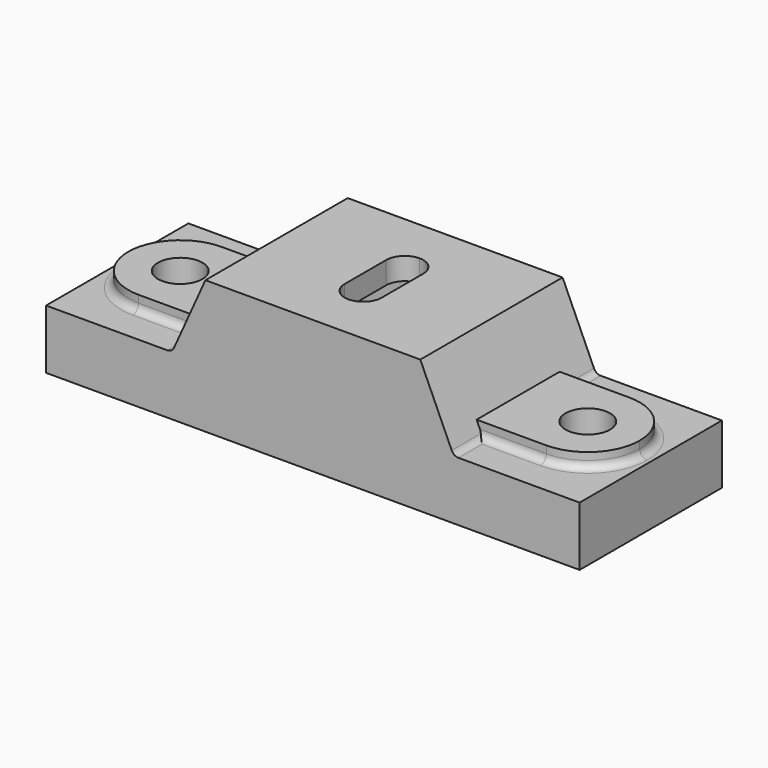
from build123d import *

# Parameters (mm, degrees)
F1_DEPTH  = 60
F3_DEPTH  = 25
F4_W      = 7.5
F4_H      = 10
F5_DEPTH  = 70
F6_R      = 34.99999
F7_R      = 5
F8_R      = 15
F9_DEPTH  = 50
F11_DEPTH = 90
F13_DEPTH = 45
F14_R     = 5


# Not quite as in the source:
# - a fillet or chamfer is up to 0.001 mm smaller than in the source, because OpenCascade refuses the exact size
# - a pattern or mirror of a feature is missing from the dataset's text; its kind, count and spacing are read off the source's solid


with BuildPart() as f1:
    # F0 (on Front) → F1 (new body, symmetric)
    with BuildSketch(Plane.XZ):
        Polygon((-180, 0), (0, 0), (180, 0), (180, 50), (90.5, 50), (72.5, 90), (0, 90), (-72.5, 90), (-90.5, 50), (-180, 50), align=None)
    extrude(amount=F1_DEPTH, both=True)

    # F2 (on face) → F3 (cut)
    with BuildSketch(Plane.XZ.offset(60)):
        Polygon((-95, 40), (-90.5, 50), (-180, 50), (-180, 40), align=None)
        Polygon((180, 50), (90.5, 50), (95, 40), (180, 40), align=None)
    f3 = extrude(amount=-F3_DEPTH, mode=Mode.SUBTRACT)

    # F3_copies: F3 across plane
    add(f3.mirror(Plane.ZX), mode=Mode.SUBTRACT)

    # F4 (on face) → F5 (cut)
    with BuildSketch(Plane.XZ.offset(35)):
        with Locations((-176.25, 45)):
            Rectangle(F4_W, F4_H)
        with Locations((176.25, 45)):
            Rectangle(F4_W, F4_H)
    extrude(amount=-F5_DEPTH, mode=Mode.SUBTRACT)

    # F6 (radius 35 in the source; OpenCascade refuses exactly that, so slightly less here)
    f6_edges = [f1.edges().sort_by_distance(p)[0] for p in [
        (172.5, -35, 45),
        (172.5, 35, 45),
        (-172.5, -35, 45),
        (-172.5, 35, 45),
    ]]
    fillet(f6_edges, radius=F6_R)

    # F7
    f7_edges = [f1.edges().sort_by_distance(p)[0] for p in [
        (116.250005, -35, 40),
        (95, -47.5, 40),
        (-116.250005, -35, 40),
        (-95, -47.5, 40),
        (-162.24874, -24.74874, 40),
        (-172.5, 0, 40),
        (-162.24874, 24.74874, 40),
        (-116.250005, 35, 40),
        (-95, 47.5, 40),
        (116.250005, 35, 40),
        (162.24874, 24.74874, 40),
        (95, 47.5, 40),
        (172.5, 0, 40),
        (162.24874, -24.74874, 40),
    ]]
    fillet(f7_edges, radius=F7_R)

    # F8 (on face) → F9 (cut)
    with BuildSketch(Plane.XY.offset(50)):
        with Locations((-137.5, 0)):
            Circle(F8_R)
        with Locations((137.5, 0)):
            Circle(F8_R)
    extrude(amount=-F9_DEPTH, mode=Mode.SUBTRACT)

    # F10 (on face) → F11 (cut)
    with BuildSketch(Plane.XY.offset(90)):
        with BuildLine():
            ThreePointArc((0, 30), (-8.8388347648, 26.3388347648), (-12.5, 17.5))
            Line((-12.5, 17.5), (-12.5, -17.5))
            ThreePointArc((-12.5, -17.5), (-8.8388347648, -26.3388347648), (0, -30))
            ThreePointArc((0, -30), (8.8388347648, -26.3388347648), (12.5, -17.5))
            Line((12.5, -17.5), (12.5, 17.5))
            ThreePointArc((12.5, 17.5), (8.8388347648, 26.3388347648), (0, 30))
        make_face()
    extrude(amount=-F11_DEPTH, mode=Mode.SUBTRACT)

    # F12 (on Front) → F13 (cut, symmetric)
    with BuildSketch(Plane.XZ):
        Polygon((-62.5, 75), (-96.25, 0), (0, 0), (96.25, 0), (62.5, 75), (0, 75), align=None)
    extrude(amount=F13_DEPTH, both=True, mode=Mode.SUBTRACT)

    # F14
    f14_edges = [f1.edges().sort_by_distance(p)[0] for p in [
        (79.375, -45, 37.5),
        (0, -45, 75),
        (62.5, 0, 75),
        (-62.5, 0, 75),
        (-79.375, -45, 37.5),
        (-79.375, 45, 37.5),
        (0, 45, 75),
        (79.375, 45, 37.5),
    ]]
    fillet(f14_edges, radius=F14_R)


solid = f1.part
